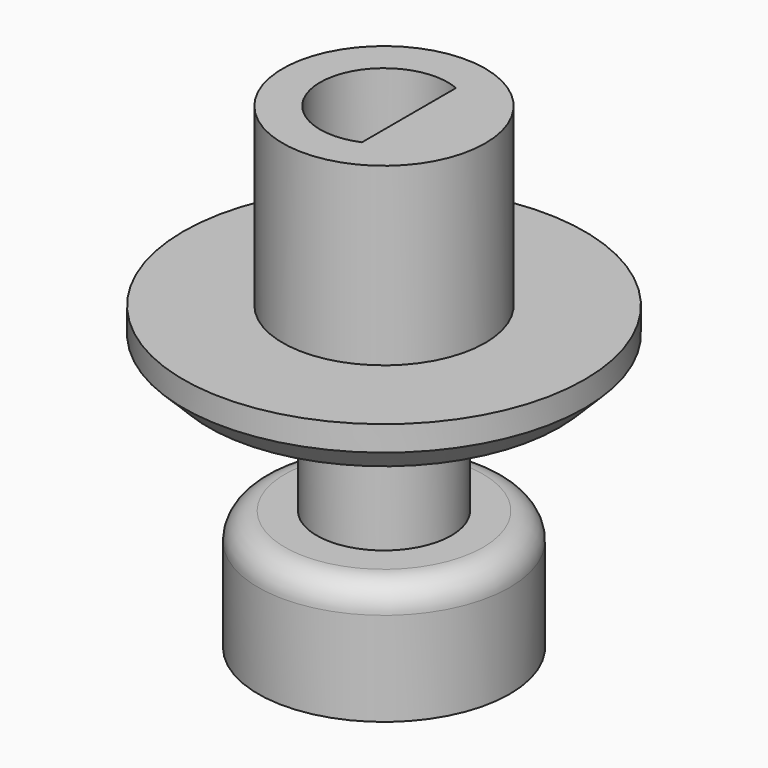
from build123d import *

# Parameters (mm, degrees)
F0_R      = 6.3637373436
F1_DEPTH  = 6.096
F2_R      = 3.4022099148
F3_DEPTH  = 12.7
F5_R      = 10.1544070979
F6_DEPTH  = 2.54
F8_R      = 5.1242922549
F9_DEPTH  = 8.89
F12_DEPTH = 7.874
F13_D     = 10.16
F13_DEPTH = 1.27
F13_TIP   = 3.0523719447
F14_R     = 1.3490625387
F15_SIZE  = 1.27


with BuildPart() as f1:
    # F0 (on Top) → F1 (new body)
    with BuildSketch(Plane.XY):
        Circle(F0_R)
    extrude(amount=F1_DEPTH)

    # F2 (on Top) → F3 (join)
    with BuildSketch(Plane.XY):
        Circle(F2_R)
    extrude(amount=F3_DEPTH)

    # F5 (on offset) → F6 (join)
    with BuildSketch(Plane.XY.offset(12.7)):
        Circle(F5_R)
    extrude(amount=F6_DEPTH)

    # F8 (on offset) → F9 (join)
    with BuildSketch(Plane.XY.offset(15.24)):
        Circle(F8_R)
    extrude(amount=F9_DEPTH)

    # F11 (on offset) → F12 (cut)
    with BuildSketch(Plane.XY.offset(24.13)):
        with BuildLine():
            Line((1.2634341, 0), (1.2634341, 2.9752182418))
            ThreePointArc((1.2634341, 2.9752182418), (-3.2323659, 0), (1.2634341, -2.9752182418))
            Line((1.2634341, -2.9752182418), (1.2634341, 0))
        make_face()
    extrude(amount=-F12_DEPTH, mode=Mode.SUBTRACT)

    # F13
    with Locations(Plane(origin=(0, 0, 0), x_dir=(1, 0, 0), z_dir=(0, 0, -1))):
        with Locations((0, 0)):
            Hole(F13_D / 2, depth=F13_DEPTH)
            with Locations((0, 0, -(F13_DEPTH + F13_TIP / 2))):  # 118° drill point
                Cone(0, F13_D / 2, F13_TIP, mode=Mode.SUBTRACT)

    # F14
    f14_edges = [f1.edges().sort_by_distance(p)[0] for p in [
        (-6.363737, 0, 6.096),
    ]]
    fillet(f14_edges, radius=F14_R)

    # F15
    f15_edges = [f1.edges().sort_by_distance(p)[0] for p in [
        (-10.154407, 0, 12.7),
    ]]
    chamfer(f15_edges, length=F15_SIZE)


solid = f1.part
